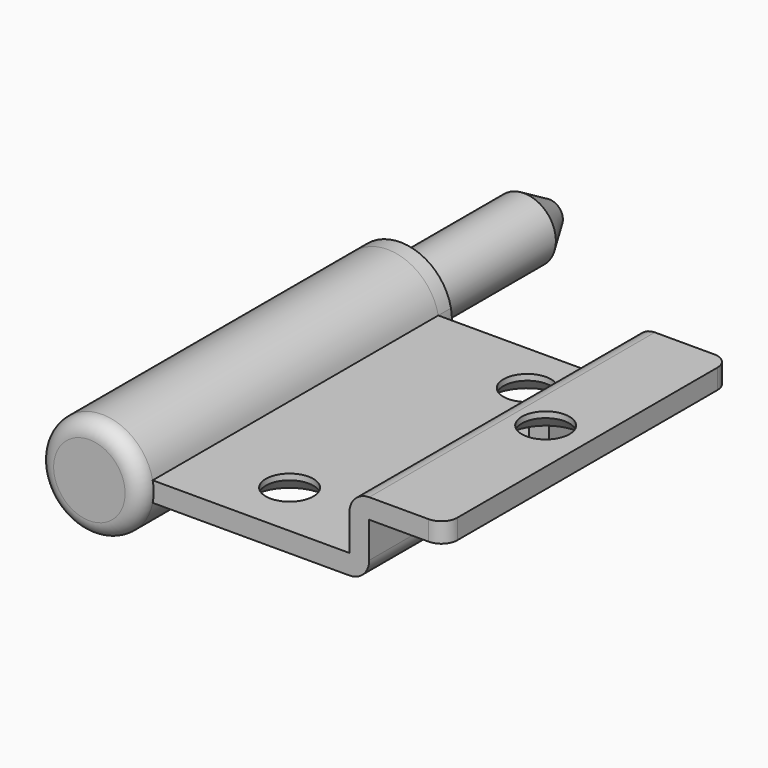
from build123d import *

# Parameters (mm, degrees)
F1_DEPTH        = 45
F2_R            = 2
F3_R            = 2.5
F5_DEPTH        = 2
F6_R            = 4
F7_DEPTH        = 23.5
F8_SIZE2        = 2.31
F8_SIZE         = 4
F10_D           = 6
F10_CSINK_D     = 9.5
F10_CSINK_ANGLE = 90
F11_R           = 6.5
F12_DEPTH       = 2
F14_W           = 5
F14_H           = 11
F15_DEPTH       = 25
F16_D           = 6
F16_CSINK_D     = 9.5
F16_CSINK_ANGLE = 90


# Not quite as in the source:
# - a fillet or chamfer that OpenCascade refuses, or shapes differently, is made with other operations: its cross-section is extruded or revolved along the edge and cut away or added
# - a feature names something its author has since deleted; it is built from what else it names


with BuildPart() as f1:
    # F0 (on Front) → F1 (new body)
    with BuildSketch(Plane.XZ):
        with BuildLine():
            Line((31.1786754111, 1.25), (6.3786754111, 1.25))
            ThreePointArc((6.3786754111, 1.25), (-6.5, 0), (6.3786754111, -1.25))
            Line((6.3786754111, -1.25), (33.6786754111, -1.25))
            Line((33.6786754111, -1.25), (33.6786754111, 5.75))
            Line((33.6786754111, 5.75), (43.1786754111, 5.75))
            Line((43.1786754111, 5.75), (43.1786754111, 8.25))
            Line((43.1786754111, 8.25), (31.1786754111, 8.25))
            Line((31.1786754111, 8.25), (31.1786754111, 1.25))
        make_face()
    extrude(amount=F1_DEPTH)

    # F2
    f2_edges = [f1.edges().sort_by_distance(p)[0] for p in [
        (43.178675, -45, 7),
        (43.178675, 0, 7),
    ]]
    fillet(f2_edges, radius=F2_R)

    # F3
    f3_edges = [f1.edges().sort_by_distance(p)[0] for p in [
        (33.678675, -22.5, -1.25),
        (31.178675, -22.5, 8.25),
    ]]
    fillet(f3_edges, radius=F3_R)

    # F4 (on face) → F5 (join)
    with BuildSketch(Plane(origin=(0, 0, 0), x_dir=(-1, 0, 0), z_dir=(0, 1, 0))):
        with BuildLine():
            ThreePointArc((-6.3786754111, -1.25), (0.6279370303, -6.469597753), (6.5, 0))
            ThreePointArc((6.5, 0), (0.6279370303, 6.469597753), (-6.3786754111, 1.25))
            ThreePointArc((-6.3786754111, 1.25), (-6.5, 0), (-6.3786754111, -1.25))
        make_face()
    extrude(amount=F5_DEPTH)

    # F6 (on face) → F7 (join)
    with BuildSketch(Plane(origin=(0, 2, 0), x_dir=(-1, 0, 0), z_dir=(0, 1, 0))):
        Circle(F6_R)
    extrude(amount=F7_DEPTH)

    # F8
    f8_edges = [f1.edges().sort_by_distance(p)[0] for p in [
        (4, 25.5, 0),
    ]]
    f8_side = f1.faces().sort_by_distance((4, 13.75, 0))[0]
    chamfer(f8_edges, length=F8_SIZE, length2=F8_SIZE2, reference=f8_side)

    # F10 (through all)
    with Locations(Plane(origin=(0, 0, -1.25), x_dir=(1, 0, 0), z_dir=(0, 0, -1))):
        with Locations((22.8786754111, 6.6), (17.8786754111, 37.8)):
            CounterSinkHole(F10_D / 2, F10_CSINK_D / 2, counter_sink_angle=F10_CSINK_ANGLE)

    # F11 (on face) → F12 (join)
    with BuildSketch(Plane.XZ.offset(45)):
        Circle(F11_R)
    extrude(amount=F12_DEPTH)

    # F13: fillet of radius 2 on 1 edges, made by hand

    # F13_s1 → F13_t2 (revolve, cut)
    with BuildSketch(Plane.XY):
        with BuildLine():
            ThreePointArc((6.5, -45), (5.9142135624, -46.4142135624), (4.5, -47))
            Line((4.5, -47), (6.5, -47))
            Line((6.5, -47), (6.5, -45))
        make_face()
    revolve(axis=Axis((0, -47, 0), (0, -1, 0)), mode=Mode.SUBTRACT)

    # F14 (on face) → F15 (cut)
    with BuildSketch(Plane(origin=(0, 0, 5.75), x_dir=(1, 0, 0), z_dir=(0, 0, -1))):
        with Locations((33.6786754111, 22.2)):
            Rectangle(F14_W, F14_H)
    extrude(amount=F15_DEPTH, mode=Mode.SUBTRACT)

    # F16 (through all)
    with Locations(Plane(origin=(0, 0, 5.75), x_dir=(1, 0, 0), z_dir=(0, 0, -1))):
        with Locations((37.6786754111, 22.2)):
            CounterSinkHole(F16_D / 2, F16_CSINK_D / 2, counter_sink_angle=F16_CSINK_ANGLE)


solid = f1.part
